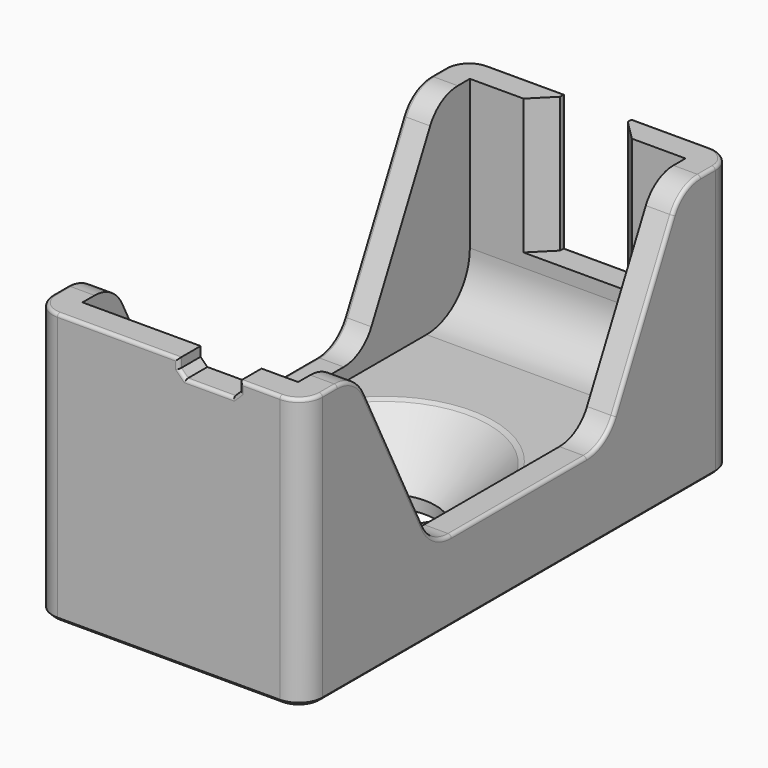
from build123d import *

# Parameters (mm, degrees)
F0_W           = 19.92
F0_H           = 39.75
F0_W_2         = 15.92
F0_H_2         = 35.75
F0_R           = 3.79
F1_DEPTH       = 5
F2_DEPTH       = 20
F4_START       = 13.8
F3_W           = 4.5
F3_H           = 2.6293848097
F4_DEPTH       = 22.1
F6_START       = 5
F5_W           = 5
F5_H           = 3
F6_DEPTH       = 15
F8_DEPTH       = 25
F9_SIZE        = 4.1
F10_R          = 1.75
F11_R          = 4
F12_T1_DEPTH   = 2
F13_SIZE       = 1.5
F14_R          = 2.847858763
F15_SIZE       = 0.25
F16_T1_DEPTH   = 9.5735533906
F16_T3_DEPTH   = 3.5535533906
F16_T5_DEPTH   = 10.6035533906
F16_T7_DEPTH   = 17.92
F16_T9_DEPTH   = 6.3135533347
F16_T11_DEPTH  = 6.3135534465
F16_T13_DEPTH  = 5
F16_T15_DEPTH  = 1.3649264893
F16_T17_DEPTH  = 1.3649264893
F16_T19_DEPTH  = 12.1323288212
F16_T21_DEPTH  = 12.1323288212
F16_T23_DEPTH  = 12.4798529787
F16_T26_ANGLE  = 90
F16_T30_DEPTH  = 1.9071067812
F16_T35_DEPTH  = 1.9142135624
F16_T41_DEPTH  = 4.7071067812
F16_T47_DEPTH  = 1.9142135624
F16_T53_DEPTH  = 1.9071067812
F16_T56_ANGLE  = 63.4349488229
F16_T58_ANGLE  = 63.4349488229
F16_T60_ANGLE  = 63.4349488229
F16_T62_ANGLE  = 63.4349488229
F16_T64_ANGLE  = 90
F16_T66_ANGLE  = 90
F16_T68_ANGLE  = 90
F16_T70_ANGLE  = 63.4349488229
F16_T72_ANGLE  = 63.4349488229
F16_T74_ANGLE  = 63.4349488229
F16_T76_ANGLE  = 63.4349488229
F16_T81_DEPTH  = 1.3035533906
F16_T85_DEPTH  = 1.9142135624
F16_T92_DEPTH  = 1.9142135624
F16_T96_DEPTH  = 4.7071067812
F16_T103_DEPTH = 4.7071067812
F16_T107_DEPTH = 1.9142135624
F16_T114_DEPTH = 1.3035533906
F16_T118_DEPTH = 1.9142135624
F16_T125_DEPTH = 10.6035533906
F16_T129_DEPTH = 5.6035533906
F16_T136_DEPTH = 5.6035533906
F16_T140_DEPTH = 10.6035533906


# Not quite as in the source:
# - a fillet or chamfer that OpenCascade refuses, or shapes differently, is made with other operations: its cross-section is extruded or revolved along the edge and cut away or added


with BuildPart() as f1:
    # F0 (on Top) → F1 (new body)
    with BuildSketch(Plane.XY):
        Rectangle(F0_W, F0_H)
        Rectangle(F0_W_2, F0_H_2, mode=Mode.SUBTRACT)
        Rectangle(F0_W_2, F0_H_2)
        Circle(F0_R, mode=Mode.SUBTRACT)
    extrude(amount=F1_DEPTH)

    # F0 (on Top) → F2 (join)
    with BuildSketch(Plane.XY):
        Rectangle(F0_W, F0_H)
        Rectangle(F0_W_2, F0_H_2, mode=Mode.SUBTRACT)
    extrude(amount=F2_DEPTH)

    # F3 (on face) → F4 (cut)
    with BuildSketch(Plane.XY.offset(5).offset(F4_START)):
        with Locations((3.01, -19.1896924049)):
            Rectangle(F3_W, F3_H)
    extrude(amount=F4_DEPTH, mode=Mode.SUBTRACT)

    # F5 (on face) → F6 (cut)
    with BuildSketch(Plane.XY.offset(5).offset(F6_START)):
        with Locations((5.59e-08, 18.7499995679)):
            Rectangle(F5_W, F5_H)
    extrude(amount=F6_DEPTH, mode=Mode.SUBTRACT)

    # F7 (on face) → F8 (cut)
    with BuildSketch(Plane(origin=(-9.96, 0, 0), x_dir=(0, -1, 0), z_dir=(-1, 0, 0))):
        Polygon((-8, 6), (0, 6), (8, 6), (15, 20), (0, 20), (-15, 20), align=None)
    extrude(amount=-F8_DEPTH, mode=Mode.SUBTRACT)

    # F9
    f9_edges = [f1.edges().sort_by_distance(p)[0] for p in [
        (-3.79, 0, 5),
    ]]
    chamfer(f9_edges, length=F9_SIZE)

    # F10
    f10_edges = [f1.edges().sort_by_distance(p)[0] for p in [
        (-9.96, 19.875, 10),
        (9.96, 19.875, 10),
        (9.96, -19.875, 10),
        (-9.96, -19.875, 10),
    ]]
    fillet(f10_edges, radius=F10_R)

    # F11
    f11_edges = [f1.edges().sort_by_distance(p)[0] for p in [
        (0, 17.875, 5),
        (0, -17.875, 5),
    ]]
    fillet(f11_edges, radius=F11_R)

    # F12: chamfer of 0.5 on 3 edges, made by hand

    # F12_s2 → F12_t1 (join)
    with BuildSketch(Plane.XZ.offset(17.875)):
        Polygon((0.76, 19.3), (1.26, 18.8), (0.76, 18.8), align=None)
        Polygon((4.76, 18.8), (5.26, 19.3), (5.26, 18.8), align=None)
    extrude(amount=F12_T1_DEPTH)


with BuildPart() as f12_tool4:
    # F12_s5 → F12_t6 (revolve)
    with BuildSketch(Plane.XZ):
        Polygon((8.0971067812, 5), (7.7435533906, 4.8535533906), (7.89, 5), align=None)
    revolve(axis=Axis((0, 0, 5), (0, 0, 1)))

    split(bisect_by=Plane.YZ.offset(7.96), keep=Keep.BOTTOM)

    split(bisect_by=Plane.YZ.offset(-7.96), keep=Keep.TOP)


with BuildPart() as f1_1:
    add(f1.part)

    # F12_t3: cut F12_tool4
    add(f12_tool4.part, mode=Mode.SUBTRACT)

    # F13
    f13_edges = [f1_1.edges().sort_by_distance(p)[0] for p in [
        (-2.5, 17.875, 15),
        (2.5, 17.875, 15),
    ]]
    chamfer(f13_edges, length=F13_SIZE)

    # F14
    f14_edges = [f1_1.edges().sort_by_distance(p)[0] for p in [
        (-8.96, -8, 6),
        (-8.96, -15, 20),
        (8.96, -15, 20),
        (8.96, -8, 6),
        (8.96, 8, 6),
        (-8.96, 8, 6),
        (-8.96, 15, 20),
        (8.96, 15, 20),
    ]]
    fillet(f14_edges, radius=F14_R)

    # F15
    f15_edges = [f1_1.edges().sort_by_distance(p)[0] for p in [
        (9.447437, -19.362437, 0),
        (9.96, 0, 0),
        (0, -19.875, 0),
        (-9.447437, -19.362437, 0),
        (-9.96, 0, 0),
        (0, 19.875, 0),
        (-9.447437, 19.362437, 0),
        (9.447437, 19.362437, 0),
    ]]
    chamfer(f15_edges, length=F15_SIZE)

    # F16: fillet of radius 0.2414213562 on 37 edges, made by hand

    # F16_s2 → F16_t1 (cut)
    with BuildSketch(Plane.YZ.offset(-8.21)):
        with BuildLine():
            ThreePointArc((-19.875, 19.7585786438), (-19.8042893219, 19.9292893219), (-19.6335786438, 20))
            Line((-19.6335786438, 20), (-19.875, 20))
            Line((-19.875, 20), (-19.875, 19.7585786438))
        make_face()
    extrude(amount=F16_T1_DEPTH, mode=Mode.SUBTRACT)

    # F16_s4 → F16_t3 (cut)
    with BuildSketch(Plane.YZ.offset(4.6564466094)):
        with BuildLine():
            ThreePointArc((-19.6335786438, 20), (-19.8042893219, 19.9292893219), (-19.875, 19.7585786438))
            Line((-19.875, 19.7585786438), (-19.875, 20))
            Line((-19.875, 20), (-19.6335786438, 20))
        make_face()
    extrude(amount=F16_T3_DEPTH, mode=Mode.SUBTRACT)

    # F16_s6 → F16_t5 (cut)
    with BuildSketch(Plane.XY.offset(10)):
        with BuildLine():
            ThreePointArc((2.7414214121, 19.875), (2.570710734, 19.8042893219), (2.5000000559, 19.6335786438))
            Line((2.5000000559, 19.6335786438), (2.5000000559, 19.875))
            Line((2.5000000559, 19.875), (2.7414214121, 19.875))
        make_face()
        with BuildLine():
            ThreePointArc((-2.7414213004, 19.875), (-2.5707106222, 19.8042893219), (-2.4999999441, 19.6335786438))
            Line((-2.4999999441, 19.6335786438), (-2.4999999441, 19.875))
            Line((-2.4999999441, 19.875), (-2.7414213004, 19.875))
        make_face()
    extrude(amount=F16_T5_DEPTH, mode=Mode.SUBTRACT)

    # F16_s8 → F16_t7 (cut)
    with BuildSketch(Plane.YZ.offset(-8.96)):
        with BuildLine():
            ThreePointArc((19.875, 0.35), (19.8566228935, 0.2576120467), (19.8042893219, 0.1792893219))
            Line((19.8042893219, 0.1792893219), (19.875, 0.25))
            Line((19.875, 0.25), (19.875, 0.35))
        make_face()
    extrude(amount=F16_T7_DEPTH, mode=Mode.SUBTRACT)

    # F16_s10 → F16_t9 (cut)
    with BuildSketch(Plane.YZ.offset(1.8964466653)):
        with BuildLine():
            ThreePointArc((19.6335786438, 20), (19.8042893219, 19.9292893219), (19.875, 19.7585786438))
            Line((19.875, 19.7585786438), (19.875, 20))
            Line((19.875, 20), (19.6335786438, 20))
        make_face()
    extrude(amount=F16_T9_DEPTH, mode=Mode.SUBTRACT)

    # F16_s12 → F16_t11 (cut)
    with BuildSketch(Plane.YZ.offset(-8.21)):
        with BuildLine():
            ThreePointArc((19.875, 19.7585786438), (19.8042893219, 19.9292893219), (19.6335786438, 20))
            Line((19.6335786438, 20), (19.875, 20))
            Line((19.875, 20), (19.875, 19.7585786438))
        make_face()
    extrude(amount=F16_T11_DEPTH, mode=Mode.SUBTRACT)

    # F16_s14 → F16_t13 (cut)
    with BuildSketch(Plane.YZ.offset(-2.4999999441)):
        with BuildLine():
            ThreePointArc((19.875, 9.7585786438), (19.8042893219, 9.9292893219), (19.6335786438, 10))
            Line((19.6335786438, 10), (19.875, 10))
            Line((19.875, 10), (19.875, 9.7585786438))
        make_face()
    extrude(amount=F16_T13_DEPTH, mode=Mode.SUBTRACT)

    # F16_s16 → F16_t15 (cut)
    with BuildSketch(Plane.XZ.offset(16.7600735107)):
        with BuildLine():
            ThreePointArc((9.96, 19.7585786438), (9.8892893219, 19.9292893219), (9.7185786438, 20))
            Line((9.7185786438, 20), (9.96, 20))
            Line((9.96, 20), (9.96, 19.7585786438))
        make_face()
        with BuildLine():
            ThreePointArc((-9.7185786438, 20), (-9.8892893219, 19.9292893219), (-9.96, 19.7585786438))
            Line((-9.96, 19.7585786438), (-9.96, 20))
            Line((-9.96, 20), (-9.7185786438, 20))
        make_face()
    extrude(amount=F16_T15_DEPTH, mode=Mode.SUBTRACT)

    # F16_s18 → F16_t17 (cut)
    with BuildSketch(Plane.XZ.offset(-18.125)):
        with BuildLine():
            ThreePointArc((9.96, 19.7585786438), (9.8892893219, 19.9292893219), (9.7185786438, 20))
            Line((9.7185786438, 20), (9.96, 20))
            Line((9.96, 20), (9.96, 19.7585786438))
        make_face()
        with BuildLine():
            ThreePointArc((-9.7185786438, 20), (-9.8892893219, 19.9292893219), (-9.96, 19.7585786438))
            Line((-9.96, 19.7585786438), (-9.96, 20))
            Line((-9.96, 20), (-9.7185786438, 20))
        make_face()
    extrude(amount=F16_T17_DEPTH, mode=Mode.SUBTRACT)

    # F16_s20 → F16_t19 (cut)
    with BuildSketch(Plane(origin=(0, -4.7871288031, 9.5742576061), x_dir=(1, 0, 0), z_dir=(0, -0.4472135955, 0.894427191))):
        with BuildLine():
            ThreePointArc((9.96, -4.7135573112), (9.8892893219, -4.5428466331), (9.7185786438, -4.472135955))
            Line((9.7185786438, -4.472135955), (9.96, -4.472135955))
            Line((9.96, -4.472135955), (9.96, -4.7135573112))
        make_face()
        with BuildLine():
            ThreePointArc((-9.96, -4.7135573112), (-9.8892893219, -4.5428466331), (-9.7185786438, -4.472135955))
            Line((-9.7185786438, -4.472135955), (-9.96, -4.472135955))
            Line((-9.96, -4.472135955), (-9.96, -4.7135573112))
        make_face()
    extrude(amount=F16_T19_DEPTH, mode=Mode.SUBTRACT)

    # F16_s22 → F16_t21 (cut)
    with BuildSketch(Plane(origin=(0, 10.2128711969, 20.4257423939), x_dir=(1, 0, 0), z_dir=(0, -0.4472135955, -0.894427191))):
        with BuildLine():
            ThreePointArc((9.96, -4.7135573112), (9.8892893219, -4.5428466331), (9.7185786438, -4.472135955))
            Line((9.7185786438, -4.472135955), (9.96, -4.472135955))
            Line((9.96, -4.472135955), (9.96, -4.7135573112))
        make_face()
        with BuildLine():
            ThreePointArc((-9.96, -4.7135573112), (-9.8892893219, -4.5428466331), (-9.7185786438, -4.472135955))
            Line((-9.7185786438, -4.472135955), (-9.96, -4.472135955))
            Line((-9.96, -4.472135955), (-9.96, -4.7135573112))
        make_face()
    extrude(amount=F16_T21_DEPTH, mode=Mode.SUBTRACT)

    # F16_s24 → F16_t23 (cut)
    with BuildSketch(Plane.XZ.offset(-6.2399264893)):
        with BuildLine():
            ThreePointArc((9.96, 5.7585786438), (9.8892893219, 5.9292893219), (9.7185786438, 6))
            Line((9.7185786438, 6), (9.96, 6))
            Line((9.96, 6), (9.96, 5.7585786438))
        make_face()
        with BuildLine():
            ThreePointArc((-9.96, 5.7585786438), (-9.8892893219, 5.9292893219), (-9.7185786438, 6))
            Line((-9.7185786438, 6), (-9.96, 6))
            Line((-9.96, 6), (-9.96, 5.7585786438))
        make_face()
    extrude(amount=F16_T23_DEPTH, mode=Mode.SUBTRACT)

    # F16_s25 → F16_t26 (revolve, cut)
    with BuildSketch(Plane.XZ.offset(18.125)):
        with BuildLine():
            ThreePointArc((-9.96, 19.7585786438), (-9.8892893219, 19.9292893219), (-9.7185786438, 20))
            Line((-9.7185786438, 20), (-9.96, 20))
            Line((-9.96, 20), (-9.96, 19.7585786438))
        make_face()
    revolve(axis=Axis((-8.21, -18.125, 20), (0, 0, 1)), revolution_arc=F16_T26_ANGLE, mode=Mode.SUBTRACT)


with BuildPart() as f16_tool28:
    # F16_s29 → F16_t30 (new body)
    with BuildSketch(Plane.XY.offset(20.6035533906)):
        with BuildLine():
            ThreePointArc((0.5185786438, -19.875), (0.6892893219, -19.8042893219), (0.76, -19.6335786438))
            Line((0.76, -19.6335786438), (0.76, -19.875))
            Line((0.76, -19.875), (0.5185786438, -19.875))
        make_face()
    extrude(amount=-F16_T30_DEPTH)

    split(bisect_by=Plane(origin=(10.03, 0, 10.03), x_dir=(0, 1, 0), z_dir=(0.7071067812, 0, 0.7071067812)), keep=Keep.TOP)


with BuildPart() as f1_2:
    add(f1_1.part)

    # F16_t27: cut F16_tool28
    add(f16_tool28.part, mode=Mode.SUBTRACT)


with BuildPart() as f16_tool33:
    # F16_s34 → F16_t35 (new body)
    with BuildSketch(Plane(origin=(-9.6967766953, 0, 9.6967766953), x_dir=(0, 1, 0), z_dir=(0.7071067812, 0, -0.7071067812))):
        with BuildLine():
            ThreePointArc((-19.875, 13.9431406744), (-19.8042893219, 14.1138513525), (-19.6335786438, 14.1845620306))
            Line((-19.6335786438, 14.1845620306), (-19.875, 14.1845620306))
            Line((-19.875, 14.1845620306), (-19.875, 13.9431406744))
        make_face()
    extrude(amount=F16_T35_DEPTH)

    split(bisect_by=Plane.YZ.offset(0.76), keep=Keep.TOP)

    split(bisect_by=Plane.XY.offset(18.8), keep=Keep.TOP)


with BuildPart() as f1_3:
    add(f1_2.part)

    # F16_t32: cut F16_tool33
    add(f16_tool33.part, mode=Mode.SUBTRACT)


with BuildPart() as f16_tool39:
    # F16_s40 → F16_t41 (new body)
    with BuildSketch(Plane.YZ.offset(0.6564466094)):
        with BuildLine():
            ThreePointArc((-19.875, 18.5585786438), (-19.8042893219, 18.7292893219), (-19.6335786438, 18.8))
            Line((-19.6335786438, 18.8), (-19.875, 18.8))
            Line((-19.875, 18.8), (-19.875, 18.5585786438))
        make_face()
    extrude(amount=F16_T41_DEPTH)

    split(bisect_by=Plane(origin=(10.03, 0, 10.03), x_dir=(0, 1, 0), z_dir=(0.7071067812, 0, 0.7071067812)), keep=Keep.TOP)

    split(bisect_by=Plane(origin=(-7.02, 0, 7.02), x_dir=(0, 1, 0), z_dir=(-0.7071067812, 0, 0.7071067812)), keep=Keep.TOP)


with BuildPart() as f1_4:
    add(f1_3.part)

    # F16_t38: cut F16_tool39
    add(f16_tool39.part, mode=Mode.SUBTRACT)


with BuildPart() as f16_tool45:
    # F16_s46 → F16_t47 (new body)
    with BuildSketch(Plane(origin=(11.3532233047, 0, 11.3532233047), x_dir=(0, 1, 0), z_dir=(0.7071067812, 0, 0.7071067812))):
        with BuildLine():
            ThreePointArc((-19.875, 9.6863578516), (-19.8042893219, 9.8570685297), (-19.6335786438, 9.9277792079))
            Line((-19.6335786438, 9.9277792079), (-19.875, 9.9277792079))
            Line((-19.875, 9.9277792079), (-19.875, 9.6863578516))
        make_face()
    extrude(amount=F16_T47_DEPTH)

    split(bisect_by=Plane.YZ.offset(5.26), keep=Keep.BOTTOM)

    split(bisect_by=Plane.XY.offset(18.8), keep=Keep.TOP)


with BuildPart() as f1_5:
    add(f1_4.part)

    # F16_t44: cut F16_tool45
    add(f16_tool45.part, mode=Mode.SUBTRACT)


with BuildPart() as f16_tool51:
    # F16_s52 → F16_t53 (new body)
    with BuildSketch(Plane.XY.offset(18.6964466094)):
        with BuildLine():
            ThreePointArc((5.5014213562, -19.875), (5.3307106781, -19.8042893219), (5.26, -19.6335786438))
            Line((5.26, -19.6335786438), (5.26, -19.875))
            Line((5.26, -19.875), (5.5014213562, -19.875))
        make_face()
    extrude(amount=F16_T53_DEPTH)

    split(bisect_by=Plane(origin=(-7.02, 0, 7.02), x_dir=(0, 1, 0), z_dir=(-0.7071067812, 0, 0.7071067812)), keep=Keep.TOP)


with BuildPart() as f1_6:
    add(f1_5.part)

    # F16_t50: cut F16_tool51
    add(f16_tool51.part, mode=Mode.SUBTRACT)

    # F16_s55 → F16_t56 (revolve, cut)
    with BuildSketch(Plane(origin=(0, -10.2128711969, 20.4257423939), x_dir=(1, 0, 0), z_dir=(0, 0.4472135955, -0.894427191))):
        with BuildLine():
            ThreePointArc((9.96, 4.7135573112), (9.8892893219, 4.5428466331), (9.7185786438, 4.472135955))
            Line((9.7185786438, 4.472135955), (9.96, 4.472135955))
            Line((9.96, 4.472135955), (9.96, 4.7135573112))
        make_face()
    revolve(axis=Axis((9.96, -16.7600735107, 17.152141237), (1, 0, 0)), revolution_arc=F16_T56_ANGLE, mode=Mode.SUBTRACT)

    # F16_s57 → F16_t58 (revolve, cut)
    with BuildSketch(Plane.XZ.offset(-16.7600735107)):
        with BuildLine():
            ThreePointArc((9.96, 19.7585786438), (9.8892893219, 19.9292893219), (9.7185786438, 20))
            Line((9.7185786438, 20), (9.96, 20))
            Line((9.96, 20), (9.96, 19.7585786438))
        make_face()
    revolve(axis=Axis((9.96, 16.7600735107, 17.152141237), (1, 0, 0)), revolution_arc=F16_T58_ANGLE, mode=Mode.SUBTRACT)

    # F16_s59 → F16_t60 (revolve, cut)
    with BuildSketch(Plane.XZ.offset(6.2399264893)):
        with BuildLine():
            ThreePointArc((9.96, 5.7585786438), (9.8892893219, 5.9292893219), (9.7185786438, 6))
            Line((9.7185786438, 6), (9.96, 6))
            Line((9.96, 6), (9.96, 5.7585786438))
        make_face()
    revolve(axis=Axis((9.96, -6.2399264893, 8.847858763), (-1, 0, 0)), revolution_arc=F16_T60_ANGLE, mode=Mode.SUBTRACT)

    # F16_s61 → F16_t62 (revolve, cut)
    with BuildSketch(Plane(origin=(0, 4.7871288031, 9.5742576061), x_dir=(1, 0, 0), z_dir=(0, 0.4472135955, 0.894427191))):
        with BuildLine():
            ThreePointArc((9.96, 4.7135573112), (9.8892893219, 4.5428466331), (9.7185786438, 4.472135955))
            Line((9.7185786438, 4.472135955), (9.96, 4.472135955))
            Line((9.96, 4.472135955), (9.96, 4.7135573112))
        make_face()
    revolve(axis=Axis((9.96, 6.2399264893, 8.847858763), (-1, 0, 0)), revolution_arc=F16_T62_ANGLE, mode=Mode.SUBTRACT)

    # F16_s63 → F16_t64 (revolve, cut)
    with BuildSketch(Plane.XZ.offset(18.125)):
        with BuildLine():
            ThreePointArc((9.96, 19.7585786438), (9.8892893219, 19.9292893219), (9.7185786438, 20))
            Line((9.7185786438, 20), (9.96, 20))
            Line((9.96, 20), (9.96, 19.7585786438))
        make_face()
    revolve(axis=Axis((8.21, -18.125, 20), (0, 0, -1)), revolution_arc=F16_T64_ANGLE, mode=Mode.SUBTRACT)

    # F16_s65 → F16_t66 (revolve, cut)
    with BuildSketch(Plane.XZ.offset(-18.125)):
        with BuildLine():
            ThreePointArc((9.96, 19.7585786438), (9.8892893219, 19.9292893219), (9.7185786438, 20))
            Line((9.7185786438, 20), (9.96, 20))
            Line((9.96, 20), (9.96, 19.7585786438))
        make_face()
    revolve(axis=Axis((8.21, 18.125, 20), (0, 0, 1)), revolution_arc=F16_T66_ANGLE, mode=Mode.SUBTRACT)

    # F16_s67 → F16_t68 (revolve, cut)
    with BuildSketch(Plane.YZ.offset(-8.21)):
        with BuildLine():
            ThreePointArc((19.875, 19.7585786438), (19.8042893219, 19.9292893219), (19.6335786438, 20))
            Line((19.6335786438, 20), (19.875, 20))
            Line((19.875, 20), (19.875, 19.7585786438))
        make_face()
    revolve(axis=Axis((-8.21, 18.125, 20), (0, 0, 1)), revolution_arc=F16_T68_ANGLE, mode=Mode.SUBTRACT)

    # F16_s69 → F16_t70 (revolve, cut)
    with BuildSketch(Plane.XZ.offset(-16.7600735107)):
        with BuildLine():
            ThreePointArc((-9.96, 19.7585786438), (-9.8892893219, 19.9292893219), (-9.7185786438, 20))
            Line((-9.7185786438, 20), (-9.96, 20))
            Line((-9.96, 20), (-9.96, 19.7585786438))
        make_face()
    revolve(axis=Axis((-9.96, 16.7600735107, 17.152141237), (1, 0, 0)), revolution_arc=F16_T70_ANGLE, mode=Mode.SUBTRACT)

    # F16_s71 → F16_t72 (revolve, cut)
    with BuildSketch(Plane.XZ.offset(16.7600735107)):
        with BuildLine():
            ThreePointArc((-9.96, 19.7585786438), (-9.8892893219, 19.9292893219), (-9.7185786438, 20))
            Line((-9.7185786438, 20), (-9.96, 20))
            Line((-9.96, 20), (-9.96, 19.7585786438))
        make_face()
    revolve(axis=Axis((-9.96, -16.7600735107, 17.152141237), (-1, 0, 0)), revolution_arc=F16_T72_ANGLE, mode=Mode.SUBTRACT)

    # F16_s73 → F16_t74 (revolve, cut)
    with BuildSketch(Plane.XZ.offset(-6.2399264893)):
        with BuildLine():
            ThreePointArc((-9.96, 5.7585786438), (-9.8892893219, 5.9292893219), (-9.7185786438, 6))
            Line((-9.7185786438, 6), (-9.96, 6))
            Line((-9.96, 6), (-9.96, 5.7585786438))
        make_face()
    revolve(axis=Axis((-9.96, 6.2399264893, 8.847858763), (1, 0, 0)), revolution_arc=F16_T74_ANGLE, mode=Mode.SUBTRACT)

    # F16_s75 → F16_t76 (revolve, cut)
    with BuildSketch(Plane(origin=(0, -4.7871288031, 9.5742576061), x_dir=(1, 0, 0), z_dir=(0, -0.4472135955, 0.894427191))):
        with BuildLine():
            ThreePointArc((-9.96, -4.7135573112), (-9.8892893219, -4.5428466331), (-9.7185786438, -4.472135955))
            Line((-9.7185786438, -4.472135955), (-9.96, -4.472135955))
            Line((-9.96, -4.472135955), (-9.96, -4.7135573112))
        make_face()
    revolve(axis=Axis((-9.96, -6.2399264893, 8.847858763), (1, 0, 0)), revolution_arc=F16_T76_ANGLE, mode=Mode.SUBTRACT)


with BuildPart() as f16_tool79:
    # F16_s80 → F16_t81 (new body)
    with BuildSketch(Plane.XY.offset(20)):
        with BuildLine():
            ThreePointArc((0.5185786438, -19.875), (0.6892893219, -19.8042893219), (0.76, -19.6335786438))
            Line((0.76, -19.6335786438), (0.76, -19.875))
            Line((0.76, -19.875), (0.5185786438, -19.875))
        make_face()
    extrude(amount=-F16_T81_DEPTH)

    split(bisect_by=Plane(origin=(10.03, 0, 10.03), x_dir=(0, 1, 0), z_dir=(-0.7071067812, 0, -0.7071067812)), keep=Keep.TOP)


with BuildPart() as f16_tool83:
    # F16_s84 → F16_t85 (new body)
    with BuildSketch(Plane(origin=(-9.6967766953, 0, 9.6967766953), x_dir=(0, 1, 0), z_dir=(0.7071067812, 0, -0.7071067812))):
        with BuildLine():
            ThreePointArc((-19.875, 13.9431406744), (-19.8042893219, 14.1138513525), (-19.6335786438, 14.1845620306))
            Line((-19.6335786438, 14.1845620306), (-19.875, 14.1845620306))
            Line((-19.875, 14.1845620306), (-19.875, 13.9431406744))
        make_face()
    extrude(amount=F16_T85_DEPTH)

    split(bisect_by=Plane.YZ.offset(0.76), keep=Keep.BOTTOM)


with BuildPart() as f16_tool79_1:
    add(f16_tool79.part)

    # F16_t87: intersect F16_tool83
    add(f16_tool83.part, mode=Mode.INTERSECT)


with BuildPart() as f1_7:
    add(f1_6.part)

    # F16_t77: cut F16_tool79
    add(f16_tool79_1.part, mode=Mode.SUBTRACT)


with BuildPart() as f16_tool90:
    # F16_s91 → F16_t92 (new body)
    with BuildSketch(Plane(origin=(-9.6967766953, 0, 9.6967766953), x_dir=(0, 1, 0), z_dir=(0.7071067812, 0, -0.7071067812))):
        with BuildLine():
            ThreePointArc((-19.875, 13.9431406744), (-19.8042893219, 14.1138513525), (-19.6335786438, 14.1845620306))
            Line((-19.6335786438, 14.1845620306), (-19.875, 14.1845620306))
            Line((-19.875, 14.1845620306), (-19.875, 13.9431406744))
        make_face()
    extrude(amount=F16_T92_DEPTH)

    split(bisect_by=Plane.XY.offset(18.8), keep=Keep.BOTTOM)


with BuildPart() as f16_tool94:
    # F16_s95 → F16_t96 (new body)
    with BuildSketch(Plane.YZ.offset(0.6564466094)):
        with BuildLine():
            ThreePointArc((-19.875, 18.5585786438), (-19.8042893219, 18.7292893219), (-19.6335786438, 18.8))
            Line((-19.6335786438, 18.8), (-19.875, 18.8))
            Line((-19.875, 18.8), (-19.875, 18.5585786438))
        make_face()
    extrude(amount=F16_T96_DEPTH)

    split(bisect_by=Plane(origin=(10.03, 0, 10.03), x_dir=(0, 1, 0), z_dir=(-0.7071067812, 0, -0.7071067812)), keep=Keep.TOP)


with BuildPart() as f16_tool90_1:
    add(f16_tool90.part)

    # F16_t98: intersect F16_tool94
    add(f16_tool94.part, mode=Mode.INTERSECT)


with BuildPart() as f1_8:
    add(f1_7.part)

    # F16_t88: cut F16_tool90
    add(f16_tool90_1.part, mode=Mode.SUBTRACT)


with BuildPart() as f16_tool101:
    # F16_s102 → F16_t103 (new body)
    with BuildSketch(Plane.YZ.offset(0.6564466094)):
        with BuildLine():
            ThreePointArc((-19.875, 18.5585786438), (-19.8042893219, 18.7292893219), (-19.6335786438, 18.8))
            Line((-19.6335786438, 18.8), (-19.875, 18.8))
            Line((-19.875, 18.8), (-19.875, 18.5585786438))
        make_face()
    extrude(amount=F16_T103_DEPTH)

    split(bisect_by=Plane(origin=(-7.02, 0, 7.02), x_dir=(0, 1, 0), z_dir=(0.7071067812, 0, -0.7071067812)), keep=Keep.TOP)


with BuildPart() as f16_tool105:
    # F16_s106 → F16_t107 (new body)
    with BuildSketch(Plane(origin=(11.3532233047, 0, 11.3532233047), x_dir=(0, 1, 0), z_dir=(0.7071067812, 0, 0.7071067812))):
        with BuildLine():
            ThreePointArc((-19.875, 9.6863578516), (-19.8042893219, 9.8570685297), (-19.6335786438, 9.9277792079))
            Line((-19.6335786438, 9.9277792079), (-19.875, 9.9277792079))
            Line((-19.875, 9.9277792079), (-19.875, 9.6863578516))
        make_face()
    extrude(amount=F16_T107_DEPTH)

    split(bisect_by=Plane.XY.offset(18.8), keep=Keep.BOTTOM)


with BuildPart() as f16_tool101_1:
    add(f16_tool101.part)

    # F16_t109: intersect F16_tool105
    add(f16_tool105.part, mode=Mode.INTERSECT)


with BuildPart() as f1_9:
    add(f1_8.part)

    # F16_t99: cut F16_tool101
    add(f16_tool101_1.part, mode=Mode.SUBTRACT)


with BuildPart() as f16_tool112:
    # F16_s113 → F16_t114 (new body)
    with BuildSketch(Plane.XY.offset(18.6964466094)):
        with BuildLine():
            ThreePointArc((5.5014213562, -19.875), (5.3307106781, -19.8042893219), (5.26, -19.6335786438))
            Line((5.26, -19.6335786438), (5.26, -19.875))
            Line((5.26, -19.875), (5.5014213562, -19.875))
        make_face()
    extrude(amount=F16_T114_DEPTH)

    split(bisect_by=Plane(origin=(-7.02, 0, 7.02), x_dir=(0, 1, 0), z_dir=(0.7071067812, 0, -0.7071067812)), keep=Keep.TOP)


with BuildPart() as f16_tool116:
    # F16_s117 → F16_t118 (new body)
    with BuildSketch(Plane(origin=(11.3532233047, 0, 11.3532233047), x_dir=(0, 1, 0), z_dir=(0.7071067812, 0, 0.7071067812))):
        with BuildLine():
            ThreePointArc((-19.875, 9.6863578516), (-19.8042893219, 9.8570685297), (-19.6335786438, 9.9277792079))
            Line((-19.6335786438, 9.9277792079), (-19.875, 9.9277792079))
            Line((-19.875, 9.9277792079), (-19.875, 9.6863578516))
        make_face()
    extrude(amount=F16_T118_DEPTH)

    split(bisect_by=Plane.YZ.offset(5.26), keep=Keep.TOP)


with BuildPart() as f16_tool112_1:
    add(f16_tool112.part)

    # F16_t120: intersect F16_tool116
    add(f16_tool116.part, mode=Mode.INTERSECT)


with BuildPart() as f1_10:
    add(f1_9.part)

    # F16_t110: cut F16_tool112
    add(f16_tool112_1.part, mode=Mode.SUBTRACT)


with BuildPart() as f16_tool123:
    # F16_s124 → F16_t125 (new body)
    with BuildSketch(Plane.XY.offset(20)):
        with BuildLine():
            ThreePointArc((2.7414214121, 19.875), (2.570710734, 19.8042893219), (2.5000000559, 19.6335786438))
            Line((2.5000000559, 19.6335786438), (2.5000000559, 19.875))
            Line((2.5000000559, 19.875), (2.7414214121, 19.875))
        make_face()
    extrude(amount=-F16_T125_DEPTH)

    split(bisect_by=Plane.XY.offset(10), keep=Keep.BOTTOM)


with BuildPart() as f16_tool127:
    # F16_s128 → F16_t129 (new body)
    with BuildSketch(Plane.YZ.offset(3.1035534465)):
        with BuildLine():
            ThreePointArc((19.875, 9.7585786438), (19.8042893219, 9.9292893219), (19.6335786438, 10))
            Line((19.6335786438, 10), (19.875, 10))
            Line((19.875, 10), (19.875, 9.7585786438))
        make_face()
    extrude(amount=-F16_T129_DEPTH)

    split(bisect_by=Plane.YZ.offset(2.5000000559), keep=Keep.TOP)


with BuildPart() as f16_tool123_1:
    add(f16_tool123.part)

    # F16_t131: intersect F16_tool127
    add(f16_tool127.part, mode=Mode.INTERSECT)


with BuildPart() as f1_11:
    add(f1_10.part)

    # F16_t121: cut F16_tool123
    add(f16_tool123_1.part, mode=Mode.SUBTRACT)


with BuildPart() as f16_tool134:
    # F16_s135 → F16_t136 (new body)
    with BuildSketch(Plane.YZ.offset(2.5000000559)):
        with BuildLine():
            ThreePointArc((19.875, 9.7585786438), (19.8042893219, 9.9292893219), (19.6335786438, 10))
            Line((19.6335786438, 10), (19.875, 10))
            Line((19.875, 10), (19.875, 9.7585786438))
        make_face()
    extrude(amount=-F16_T136_DEPTH)

    split(bisect_by=Plane.YZ.offset(-2.4999999441), keep=Keep.BOTTOM)


with BuildPart() as f16_tool138:
    # F16_s139 → F16_t140 (new body)
    with BuildSketch(Plane.XY.offset(9.3964466094)):
        with BuildLine():
            ThreePointArc((-2.7414213004, 19.875), (-2.5707106222, 19.8042893219), (-2.4999999441, 19.6335786438))
            Line((-2.4999999441, 19.6335786438), (-2.4999999441, 19.875))
            Line((-2.4999999441, 19.875), (-2.7414213004, 19.875))
        make_face()
    extrude(amount=F16_T140_DEPTH)

    split(bisect_by=Plane.XY.offset(10), keep=Keep.BOTTOM)


with BuildPart() as f16_tool134_1:
    add(f16_tool134.part)

    # F16_t142: intersect F16_tool138
    add(f16_tool138.part, mode=Mode.INTERSECT)


with BuildPart() as f1_12:
    add(f1_11.part)

    # F16_t132: cut F16_tool134
    add(f16_tool134_1.part, mode=Mode.SUBTRACT)


solid = f1_12.part
